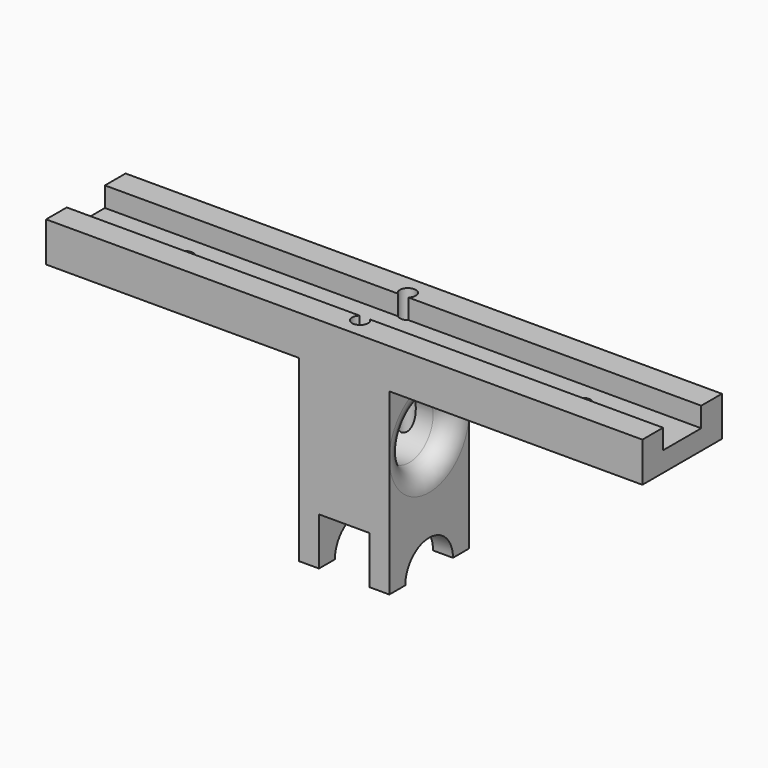
from build123d import *

# Parameters (mm, degrees)
F0_W     = 150
F0_H     = 25
F0_R     = 2
F1_DEPTH = 55
F2_W     = 12
F2_H     = 5
F3_DEPTH = 150.001
F4_W     = 63.65
F4_H     = 45
F4_W_2   = 12.7
F4_H_2   = 12
F5_DEPTH = 25.001
F7_DEPTH = 86.351
F6_R     = 7.5
F8_DEPTH = 86.351
F9_R     = 4.99999
F10_SIZE = 1.5


# Not quite as in the source:
# - a fillet or chamfer is up to 0.001 mm smaller than in the source, because OpenCascade refuses the exact size


with BuildPart() as f1:
    # F0 (on Top) → F1 (new body)
    with BuildSketch(Plane.XY):
        Rectangle(F0_W, F0_H)
        with Locations((0, -7.5)):
            Circle(F0_R, mode=Mode.SUBTRACT)
        with Locations((-50, 0)):
            Circle(F0_R, mode=Mode.SUBTRACT)
        with Locations((50, 0)):
            Circle(F0_R, mode=Mode.SUBTRACT)
        with Locations((0, 7.5)):
            Circle(F0_R, mode=Mode.SUBTRACT)
    extrude(amount=F1_DEPTH)

    # F2 (on face) → F3 (cut, through all)
    with BuildSketch(Plane.YZ.offset(75)):
        with Locations((0, 52.5)):
            Rectangle(F2_W, F2_H)
    extrude(amount=-F3_DEPTH, mode=Mode.SUBTRACT)

    # F4 (on face) → F5 (cut, through all)
    with BuildSketch(Plane.XZ.offset(12.5)):
        with Locations((43.175, 22.5)):
            Rectangle(F4_W, F4_H)
        with Locations((-43.175, 22.5)):
            Rectangle(F4_W, F4_H)
        with Locations((0, 6)):
            Rectangle(F4_W_2, F4_H_2)
    extrude(amount=-F5_DEPTH, mode=Mode.SUBTRACT)

    # F6 (on face) → F7 (cut, through all)
    with BuildSketch(Plane(origin=(-11.35, 0, 0), x_dir=(0, -1, 0), z_dir=(-1, 0, 0))):
        with BuildLine():
            Line((-7.5, 0), (7.5, 0))
            ThreePointArc((7.5, 0), (0, 7.5), (-7.5, 0))
        make_face()
    extrude(amount=-F7_DEPTH, mode=Mode.SUBTRACT)

    # F6 (on face) → F8 (cut, through all)
    with BuildSketch(Plane(origin=(-11.35, 0, 0), x_dir=(0, -1, 0), z_dir=(-1, 0, 0))):
        with Locations((0, 30)):
            Circle(F6_R)
    extrude(amount=-F8_DEPTH, mode=Mode.SUBTRACT)

    # F9 (radius 5 in the source; OpenCascade refuses exactly that, so slightly less here)
    f9_edges = [f1.edges().sort_by_distance(p)[0] for p in [
        (-11.35, 7.5, 30),
        (11.35, 7.5, 30),
    ]]
    fillet(f9_edges, radius=F9_R)

    # F10
    f10_edges = [f1.edges().sort_by_distance(p)[0] for p in [
        (48, 0, 45),
        (-52, 0, 45),
    ]]
    chamfer(f10_edges, length=F10_SIZE)


solid = f1.part
